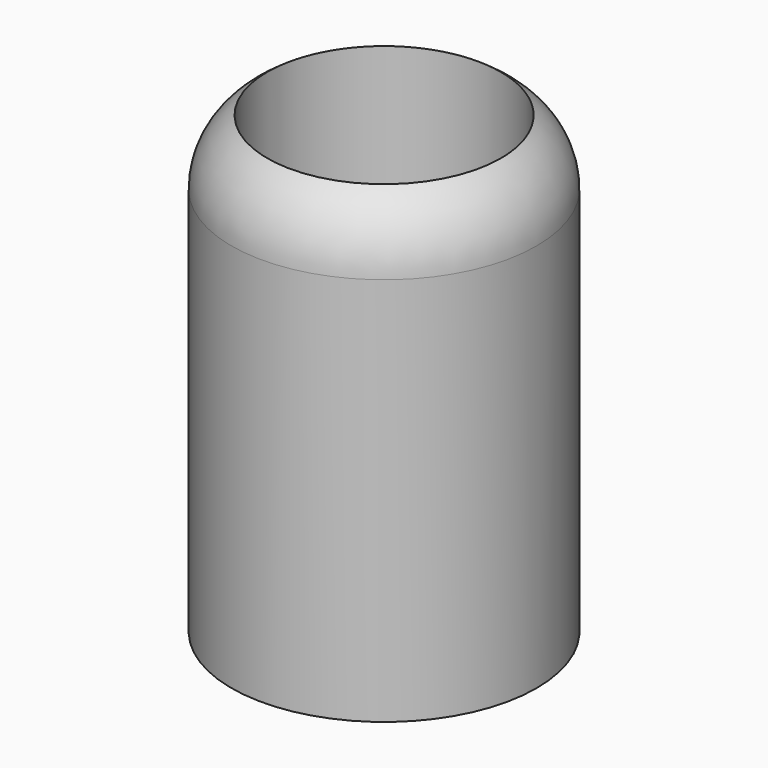
from build123d import *

# Parameters (mm, degrees)
F0_R     = 49.7765250683
F1_DEPTH = 152.4
F2_R     = 25.4
F4_D     = 76.2


# Not quite as in the source:
# - the program builds the solid bodies; features that only make, move or delete a surface that nothing else refers to are left out


with BuildPart() as f1:
    # F0 (on Top) → F1 (new body)
    with BuildSketch(Plane.XY):
        Circle(F0_R)
    extrude(amount=F1_DEPTH)

    # F2
    f2_edges = [f1.edges().sort_by_distance(p)[0] for p in [
        (-49.776525, 0, 152.4),
    ]]
    fillet(f2_edges, radius=F2_R)

    # F4 (through all)
    with Locations(Plane.XY.offset(152.4)):
        with Locations((0, 0)):
            Hole(F4_D / 2)


solid = f1.part
